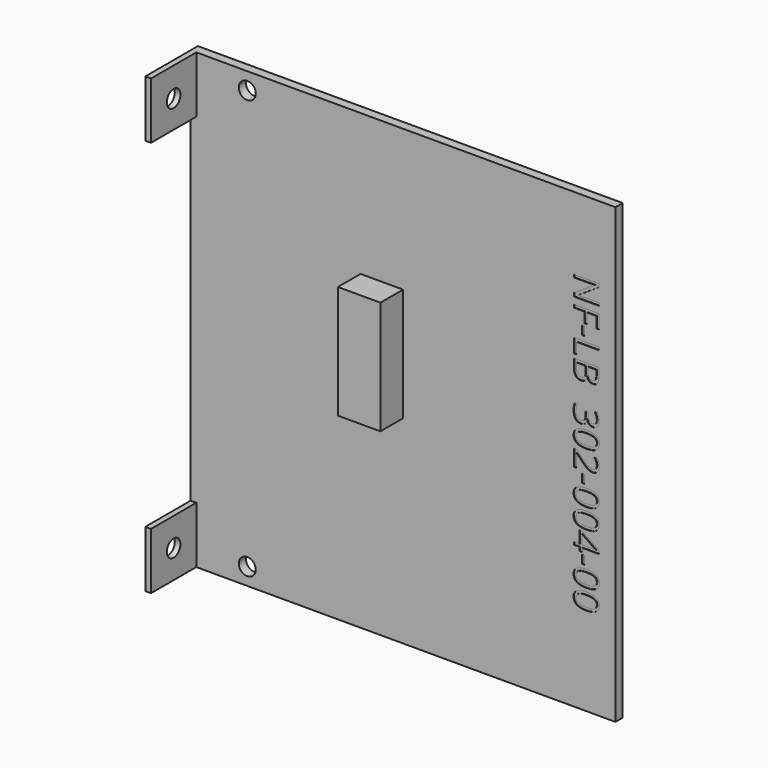
from build123d import *

# Parameters (mm, degrees)
F0_R         = 1.5
F0_W         = 7.5
F0_H         = 20
F0_W_2       = 1
F0_H_2       = 10
F1_DEPTH     = 1.6
F2_DEPTH     = 5
F3_TEXT_SIZE = 6.1743944469
F4_DEPTH     = 0.1
F5_DEPTH     = 10
F6_R         = 1.5
F7_DEPTH     = 1


# Not quite as in the source:
# - Text() gives the source's letters only with a copy of the font that has no kerning and outlines rounded to 1/6400 em; it was checked with that copy


with BuildPart() as f1:
    # F0 (on Front) → F1 (new body)
    with BuildSketch(Plane.XZ):
        Polygon((-36.5, -40), (37.5, -40), (37.5, 40), (-36.5, 40), (-36.5, 30), (-37.5, 30), (-37.5, -30), (-36.5, -30), align=None)
        with Locations((-27.5, -37)):
            Circle(F0_R, mode=Mode.SUBTRACT)
        with Locations((-3.75, 5)):
            Rectangle(F0_W, F0_H, mode=Mode.SUBTRACT)
        with Locations((-27.5, 37)):
            Circle(F0_R, mode=Mode.SUBTRACT)
        with Locations((-3.75, 5)):
            Rectangle(F0_W, F0_H)
        with Locations((-37, -35)):
            Rectangle(F0_W_2, F0_H_2)
        with Locations((-37, 35)):
            Rectangle(F0_W_2, F0_H_2)
    extrude(amount=-F1_DEPTH)

    # F0 (on Front) → F2 (join)
    with BuildSketch(Plane.XZ):
        with Locations((-3.75, 5)):
            Rectangle(F0_W, F0_H)
    extrude(amount=F2_DEPTH)

    # F3 (on face) → F4 (cut)
    with BuildSketch(Plane.XZ):
        with Locations(Location((30.1700662822, 27.7718417346), (0, 0, -90))):
            Text('NF-LB  302-004-00', F3_TEXT_SIZE, font='Open Sans', text_align=(TextAlign.LEFT, TextAlign.BOTTOM))
    extrude(amount=-F4_DEPTH, mode=Mode.SUBTRACT)

    # F0 (on Front) → F5 (join)
    with BuildSketch(Plane.XZ):
        with Locations((-37, 35)):
            Rectangle(F0_W_2, F0_H_2)
        with Locations((-37, -35)):
            Rectangle(F0_W_2, F0_H_2)
    extrude(amount=F5_DEPTH)

    # F6 (on face) → F7 (cut, through all)
    with BuildSketch(Plane(origin=(-37.5, 0, 0), x_dir=(0, -1, 0), z_dir=(-1, 0, 0))):
        with Locations((5, -35.0045712793)):
            Circle(F6_R)
        with Locations((5, 34.8643921316)):
            Circle(F6_R)
    extrude(amount=-F7_DEPTH, mode=Mode.SUBTRACT)


solid = f1.part
